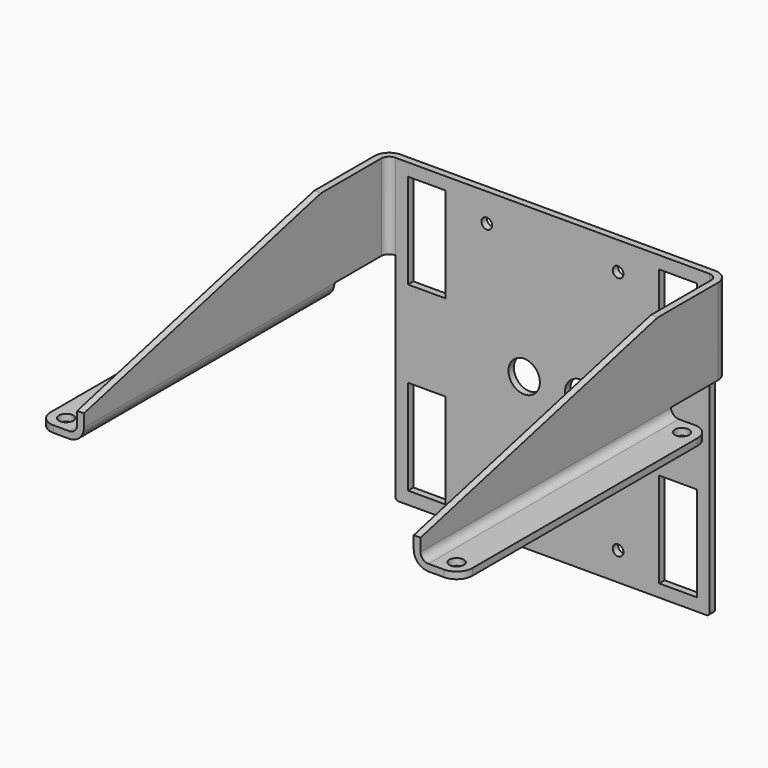
from build123d import *

# Parameters (mm, degrees)
F1_DEPTH  = 21.70684
F2_W      = 1.70942
F2_H      = 79.1155667
F3_DEPTH  = 3.69316
F4_W      = 9.92124
F4_H      = 1.70942
F5_DEPTH  = 79.1155667
F6_W      = 79.3829248
F6_H      = 1.70942
F7_DEPTH  = 54.49316
F8_W      = 9.5329248
F8_H      = 24
F8_R      = 1.35255
F8_R_2    = 3.96875
F9_DEPTH  = 1.70942
F10_R     = 0.762
F11_R     = 3.96875
F12_R     = 3.69316
F13_R     = 1.98374
F15_DEPTH = 86.7692448
F16_R     = 1.8288
F17_DEPTH = 1.70942


with BuildPart() as f1:
    # F0 (on Top) → F1 (new body)
    with BuildSketch(Plane.XY):
        Polygon((-1.70942, -95.9058534), (0, -95.9058534), (0, 0), (83.3504048, 0), (83.3504048, -95.9058534), (85.0598248, -95.9058534), (85.0598248, 1.70942), (-1.70942, 1.70942), align=None)
    extrude(amount=F1_DEPTH)

    # F2 (on face) → F3 (join)
    with BuildSketch(Plane(origin=(0, 0, 0), x_dir=(1, 0, 0), z_dir=(0, 0, -1))):
        with Locations((-0.85471, 56.34807005)):
            Rectangle(F2_W, F2_H)
        with Locations((84.2051148, 56.34807005)):
            Rectangle(F2_W, F2_H)
    extrude(amount=F3_DEPTH)

    # F4 (on face) → F5 (join, through all)
    with BuildSketch(Plane.XZ.offset(95.9058534)):
        with Locations((90.0204448, -2.83845)):
            Rectangle(F4_W, F4_H)
        with Locations((-6.67004, -2.83845)):
            Rectangle(F4_W, F4_H)
    extrude(amount=-F5_DEPTH)

    # F6 (on face) → F7 (join)
    with BuildSketch(Plane(origin=(0, 0, 0), x_dir=(1, 0, 0), z_dir=(0, 0, -1))):
        with Locations((41.6752024, -0.85471)):
            Rectangle(F6_W, F6_H)
    extrude(amount=F7_DEPTH)

    # F8 (on face) → F9 (cut, through all)
    with BuildSketch(Plane(origin=(0, 1.70942, 0), x_dir=(-1, 0, 0), z_dir=(0, 1, 0))):
        with Locations((-9.9252024, -39.31816)):
            Rectangle(F8_W, F8_H)
        with Locations((-9.9252024, 6.53184)):
            Rectangle(F8_W, F8_H)
        with Locations((-73.4252024, 6.53184)):
            Rectangle(F8_W, F8_H)
        with Locations((-73.4252024, -39.31816)):
            Rectangle(F8_W, F8_H)
        with Locations((-25.0871228, -47.34941)):
            Circle(F8_R)
        with Locations((-58.263282, -47.34941)):
            Circle(F8_R)
        with Locations((-58.263282, 14.56309)):
            Circle(F8_R)
        with Locations((-25.0871228, 14.56309)):
            Circle(F8_R)
        with Locations((-48.8189524, -16.39316)):
            Circle(F8_R_2)
        with Locations((-34.5314524, -16.39316)):
            Circle(F8_R_2)
    extrude(amount=-F9_DEPTH, mode=Mode.SUBTRACT)

    # F10
    f10_edges = [f1.edges().sort_by_distance(p)[0] for p in [
        (1.98374, 0.85471, -54.49316),
        (81.366665, 0.85471, -54.49316),
    ]]
    fillet(f10_edges, radius=F10_R)

    # F11
    f11_edges = [f1.edges().sort_by_distance(p)[0] for p in [
        (94.981065, -95.905853, -2.83845),
        (-11.63066, -16.790287, -2.83845),
        (-11.63066, -95.905853, -2.83845),
        (94.981065, -16.790287, -2.83845),
    ]]
    fillet(f11_edges, radius=F11_R)

    # F12
    f12_edges = [f1.edges().sort_by_distance(p)[0] for p in [
        (0, -56.34807, -3.69316),
        (-1.70942, 1.70942, 10.85342),
        (85.059825, 1.70942, 10.85342),
        (83.350405, -56.34807, -3.69316),
    ]]
    fillet(f12_edges, radius=F12_R)

    # F13
    f13_edges = [f1.edges().sort_by_distance(p)[0] for p in [
        (83.350405, 0, 10.85342),
        (0, 0, 10.85342),
        (85.059825, -56.34807, -1.98374),
        (-1.70942, -56.34807, -1.98374),
    ]]
    fillet(f13_edges, radius=F13_R)

    # F14 (on face) → F15 (cut, through all)
    with BuildSketch(Plane(origin=(-1.70942, 0, 0), x_dir=(0, -1, 0), z_dir=(-1, 0, 0))):
        Polygon((95.9058534, 21.70684), (21.03374, 21.70684), (95.9058534, 3.175), align=None)
    extrude(amount=-F15_DEPTH, mode=Mode.SUBTRACT)

    # F16 (on face) → F17 (cut, through all)
    with BuildSketch(Plane(origin=(0, 0, -3.69316), x_dir=(1, 0, 0), z_dir=(0, 0, -1))):
        with Locations((-7.66191, 91.9371034)):
            Circle(F16_R)
        with Locations((-7.66191, 20.7590367)):
            Circle(F16_R)
        with Locations((91.0123148, 91.9371034)):
            Circle(F16_R)
        with Locations((91.0123148, 20.7590367)):
            Circle(F16_R)
    extrude(amount=-F17_DEPTH, mode=Mode.SUBTRACT)


solid = f1.part
